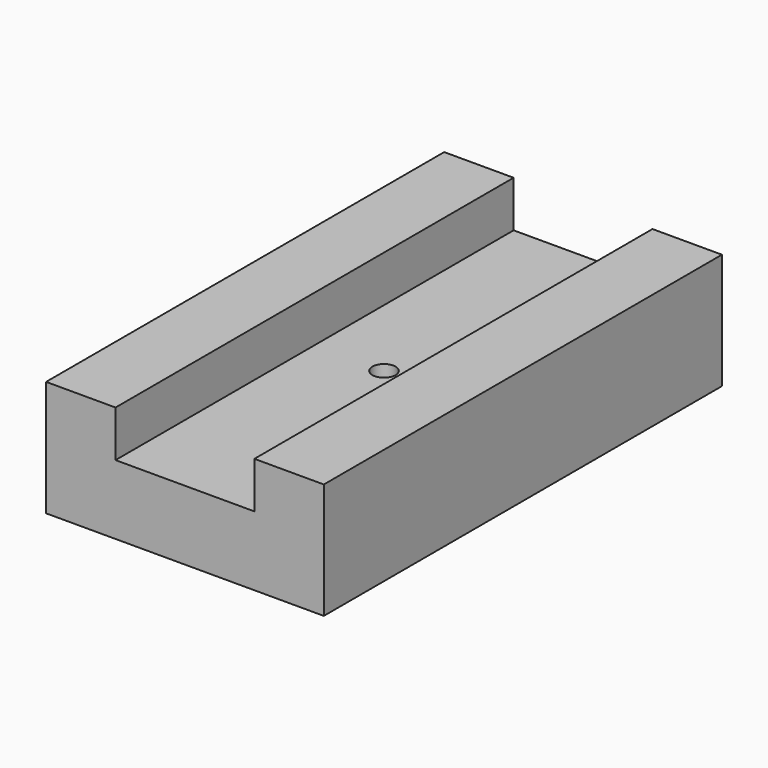
from build123d import *

# Parameters (mm, degrees)
F0_W           = 76.2
F0_H           = 136.525
F1_DEPTH       = 19.05
F2_W           = 19.05
F2_H           = 12.7
F3_DEPTH       = 136.525
F5_D           = 6.35
F5_CBORE_D     = 19.05
F5_CBORE_DEPTH = 12.7


# Not quite as in the source:
# - a length typed as a fraction of an inch, garbled in the dataset ("3 / 203.2 mm" for 3/8 in), is restored


with BuildPart() as f1:
    # F0 (on Top) → F1 (new body)
    with BuildSketch(Plane.XY):
        Rectangle(F0_W, F0_H)
    extrude(amount=F1_DEPTH)

    # F2 (on face) → F3 (join)
    with BuildSketch(Plane.XZ.offset(68.2625)):
        with Locations((-28.575, 25.4)):
            Rectangle(F2_W, F2_H)
        with Locations((28.575, 25.4)):
            Rectangle(F2_W, F2_H)
    extrude(amount=-F3_DEPTH)

    # F5 (through all)
    with Locations(Plane(origin=(0, 0, 0), x_dir=(1, 0, 0), z_dir=(0, 0, -1))):
        with Locations((0, 0)):
            CounterBoreHole(F5_D / 2, F5_CBORE_D / 2, F5_CBORE_DEPTH)


solid = f1.part
